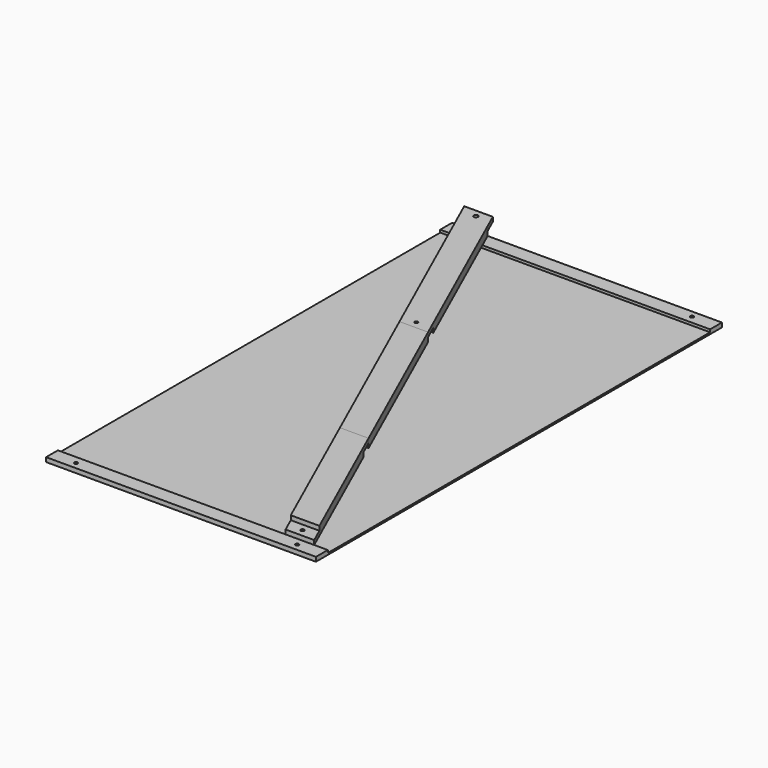
from build123d import *

# Parameters (mm, degrees)
F0_W      = 310
F0_H      = 17
F0_R      = 2
F1_DEPTH  = 5
F0_H_2    = 549
F2_DEPTH  = 2
F4_DEPTH  = 10
F3_R      = 2
F6_DEPTH  = 5
F8_DEPTH  = 5
F9_R      = 2
F10_DEPTH = 25
F12_START = -5
F12_DEPTH = 5
F13_DEPTH = 10
F14_DEPTH = 5
F15_R     = 2.4432897083
F16_DEPTH = 25
F17_R     = 1.8572425824
F18_DEPTH = 25


# Not quite as in the source:
# - a feature names something its author has since deleted; it is built from what else it names


with BuildPart() as f1:
    # F0 (on Top) → F1 (new body)
    with BuildSketch(Plane.XY):
        with Locations((8.0607275963, 283.7472317666)):
            Rectangle(F0_W, F0_H)
        with Locations((-118.9392724037, 284.2472317666)):
            Circle(F0_R, mode=Mode.SUBTRACT)
        with Locations((135.0607275963, 284.2472317666)):
            Circle(F0_R, mode=Mode.SUBTRACT)
    extrude(amount=F1_DEPTH)



with BuildPart() as f1b:
    # F0 (on Top) → F1, piece 2 (new body)
    with BuildSketch(Plane.XY):
        with Locations((8.0607275963, -282.2527682334)):
            Rectangle(F0_W, F0_H)
        with Locations((-118.9392724037, -282.7527682334)):
            Circle(F0_R, mode=Mode.SUBTRACT)
        with Locations((135.0607275963, -282.7527682334)):
            Circle(F0_R, mode=Mode.SUBTRACT)
    extrude(amount=F1_DEPTH)


with BuildPart() as f1_1:
    add(f1.part)

    add(f1b.part)  # F2 merges F1b
    # F0 (on Top) → F2 (join)
    with BuildSketch(Plane.XY):
        with Locations((8.0607275963, 0.7472317666)):
            Rectangle(F0_W, F0_H_2)
    extrude(amount=F2_DEPTH)

    # F11 (on face) → F14 (cut)
    with BuildSketch(Plane.XY.offset(15)):
        Polygon((-19.030874229, 97.9138984332), (-26.6463945112, 114.9138984332), (-59.5190403609, 114.9138984332), (-51.9035200787, 97.9138984332), align=None)
        Polygon((-95.7537963986, 309.2138984332), (-113.6873116188, 309.2138984332), (-106.0740024037, 292.2188341618), (-95.7537963986, 292.2188341618), align=None)
        Polygon((-106.0740024037, 292.2188341618), (-113.6873116188, 309.2138984332), (-146.5599574685, 309.2138984332), (-138.9466482534, 292.2188341618), align=None)
        Polygon((-138.9466482534, 292.2188341618), (-146.5599574685, 309.2138984332), (-168.3874875307, 309.2138984332), (-168.3874875307, 292.2188341618), align=None)
    extrude(amount=F14_DEPTH, mode=Mode.SUBTRACT)


with BuildPart() as f4:
    # F3 (on face) → F4 (new body)
    with BuildSketch(Plane.XY.offset(5)):
        Polygon((147.4554403895, -273.7307487662), (114.5827945397, -273.7307487662), (114.6075910324, -273.7861015668), (147.4802368821, -273.7861015668), align=None)
        Polygon((68.0249752713, -96.4194349001), (35.1523294216, -96.4194349001), (114.5827945397, -273.7307487662), (147.4554403895, -273.7307487662), align=None)
    extrude(amount=F4_DEPTH)

    # F5 (on face) → F6 (cut)
    with BuildSketch(Plane.XY.offset(15)):
        Polygon((114.6075910324, -273.7861015668), (147.4802368821, -273.7861015668), (139.8647165999, -256.7861015668), (106.9920707502, -256.7861015668), align=None)
    extrude(amount=-F6_DEPTH, mode=Mode.SUBTRACT)

    # F7 (on face) → F8 (cut)
    with BuildSketch(Plane.XY.offset(5)):
        Polygon((68.0249752713, -96.4194349001), (35.1523294216, -96.4194349001), (42.7678497038, -113.4194349001), (75.6404955535, -113.4194349001), align=None)
    extrude(amount=F8_DEPTH, mode=Mode.SUBTRACT)

    # F9 (on face) → F10 (cut)
    with BuildSketch(Plane.XY.offset(10)):
        with Locations((127.2361538162, -265.2861015668)):
            Circle(F9_R)
    extrude(amount=-F10_DEPTH, mode=Mode.SUBTRACT)


with BuildPart() as f4b:
    # F3 (on face) → F4, piece 2 (new body)
    with BuildSketch(Plane.XY.offset(5)):
        Polygon((-131.3438492968, 275.2472317666), (-51.9035200787, 97.9138984332), (-19.030874229, 97.9138984332), (-98.4712034471, 275.2472317666), align=None)
        Polygon((-138.959369579, 292.2472317666), (-131.3438492968, 275.2472317666), (-98.4712034471, 275.2472317666), (-106.0867237293, 292.2472317666), align=None)
        with Locations((-118.9392724037, 284.2472317666)):
            Circle(F3_R, mode=Mode.SUBTRACT)
        Polygon((-146.5599574685, 309.2138984332), (-138.959369579, 292.2472317666), (-106.0867237293, 292.2472317666), (-113.6873116188, 309.2138984332), align=None)
        with Locations((-118.9392724037, 284.2472317666)):
            Circle(F3_R)
    extrude(amount=F4_DEPTH)

    # F11 (on face) → F12 (cut)
    with BuildSketch(Plane.XY.offset(15).offset(F12_START)):
        Polygon((-19.030874229, 97.9138984332), (-26.6463945112, 114.9138984332), (-59.5190403609, 114.9138984332), (-51.9035200787, 97.9138984332), align=None)
        Polygon((-106.0740024037, 292.2188341618), (-113.6873116188, 309.2138984332), (-146.5599574685, 309.2138984332), (-138.9466482534, 292.2188341618), align=None)
    extrude(amount=-F12_DEPTH, mode=Mode.SUBTRACT)

    # F15 (on face) → F16 (cut)
    with BuildSketch(Plane(origin=(0, 0, 10), x_dir=(1, 0, 0), z_dir=(0, 0, -1))):
        with Locations((-126.3180854696, -300.7188341618)):
            Circle(F15_R)
    extrude(amount=-F16_DEPTH, mode=Mode.SUBTRACT)

    # F17 (on face) → F18 (cut)
    with BuildSketch(Plane(origin=(0, 0, 10), x_dir=(1, 0, 0), z_dir=(0, 0, -1))):
        with Locations((-39.274957295, -106.4138984332)):
            Circle(F17_R)
    extrude(amount=-F18_DEPTH, mode=Mode.SUBTRACT)


with BuildPart() as f13:
    # F3 (on face) → F13 (new body)
    with BuildSketch(Plane.XY.offset(5)):
        Polygon((-19.030874229, 97.9138984332), (-51.9035200787, 97.9138984332), (35.1523294216, -96.4194349001), (68.0249752713, -96.4194349001), align=None)
    extrude(amount=F13_DEPTH)


solid = Compound([f1_1.part, f4.part, f4b.part, f13.part])
